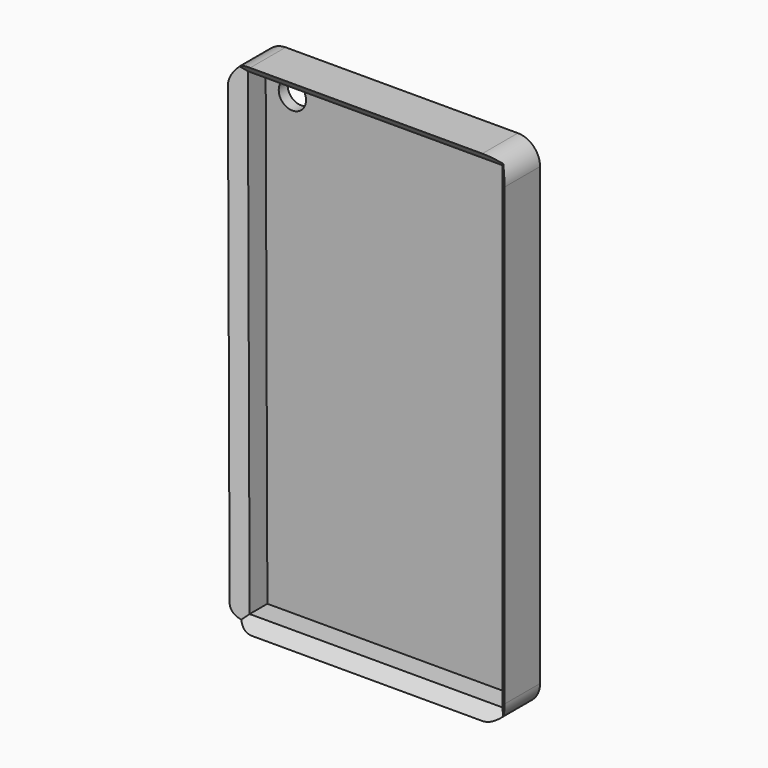
from build123d import *

# Parameters (mm, degrees)
F1_DEPTH     = 12.7
F2_T         = -2.54
F3_R         = 5.08
F4_T1_DEPTH  = 109.2192415341
F4_T6_DEPTH  = 70.8878458195
F4_T11_DEPTH = 71.2857341695
F4_T16_DEPTH = 135.3482654479
F4_T23_DEPTH = 70.8878458195
F4_S24_R     = 5.08
F4_T25_DEPTH = 37
F4_T29_DEPTH = 135.3482654479
F4_S30_R     = 5.08
F4_T31_DEPTH = 69
F4_T38_DEPTH = 122.283391113
F4_S39_R     = 5.08
F4_T40_DEPTH = 63
F4_T44_DEPTH = 83.9519953984
F4_S45_R     = 5.08
F4_T46_DEPTH = 44
F4_T53_DEPTH = 84.3498837483
F4_S54_R     = 5.08
F4_T55_DEPTH = 44
F4_T59_DEPTH = 122.283391113
F4_S60_R     = 5.08
F4_T61_DEPTH = 63
F4_T68_DEPTH = 71.2857341695
F4_S69_R     = 5.08
F4_T70_DEPTH = 37
F4_T74_DEPTH = 135.3482654479
F4_S75_R     = 5.08
F4_T76_DEPTH = 69
F5_R         = 3.1205414485
F6_DEPTH     = 25.4


# Not quite as in the source:
# - a fillet or chamfer that OpenCascade refuses, or shapes differently, is made with other operations: its cross-section is extruded or revolved along the edge and cut away or added


with BuildPart() as f1:
    # F0 (on Front) → F1 (new body)
    with BuildSketch(Plane.XZ):
        Polygon((-76.0919898748, 56.9143295288), (-75.6755949615, -57.3849120053), (-12.7811351476, -57.3849120053), (-12.7811351476, 56.9143295288), align=None)
    extrude(amount=F1_DEPTH)

    # F2
    f2_openings = [f1.faces().sort_by_distance(p)[0] for p in [
        (-44.332578, -12.7, -0.172439),
    ]]
    offset(amount=F2_T, openings=f2_openings)

    # F3
    f3_edges = [f1.edges().sort_by_distance(p)[0] for p in [
        (-12.781135, -6.35, 56.91433),
        (-76.09199, -6.35, 56.91433),
        (-12.781135, -6.35, -57.384912),
        (-75.675595, -6.35, -57.384912),
    ]]
    fillet(f3_edges, radius=F3_R)

    # F4: chamfer of 5.08 on 4 edges, made by hand

    # F4_s2 → F4_t1 (cut)
    with BuildSketch(Plane.XY.offset(-54.8449120053)):
        Polygon((-10.2411351476, -12.7), (-15.3211351476, -7.62), (-15.3211351476, -12.7), align=None)
    extrude(amount=F4_T1_DEPTH, mode=Mode.SUBTRACT)


with BuildPart() as f4_tool4:
    # F4_s5 → F4_t6 (new body)
    with BuildSketch(Plane.YZ.offset(-86.2089809671)):
        Polygon((-12.7, -59.9249120053), (-7.62, -54.8449120053), (-12.7, -54.8449120053), align=None)
    extrude(amount=F4_T6_DEPTH)

    split(bisect_by=Plane(origin=(-73.3436593453, 0, -0.2671927326), x_dir=(0, 1, 0), z_dir=(0.9999933643, 0, 0.0036430001)), keep=Keep.TOP)


with BuildPart() as f1_1:
    add(f1.part)

    # F4_t3: cut F4_tool4
    add(f4_tool4.part, mode=Mode.SUBTRACT)


with BuildPart() as f4_tool9:
    # F4_s10 → F4_t11 (new body)
    with BuildSketch(Plane.YZ.offset(-15.3211351476)):
        Polygon((-12.7, 59.4543295288), (-7.62, 54.3743295288), (-12.7, 54.3743295288), align=None)
    extrude(amount=-F4_T11_DEPTH)

    split(bisect_by=Plane(origin=(-73.3436593453, 0, -0.2671927326), x_dir=(0, 1, 0), z_dir=(0.9999933643, 0, 0.0036430001)), keep=Keep.TOP)


with BuildPart() as f1_2:
    add(f1_1.part)

    # F4_t8: cut F4_tool9
    add(f4_tool9.part, mode=Mode.SUBTRACT)


with BuildPart() as f4_tool14:
    # F4_s15 → F4_t16 (new body)
    with BuildSketch(Plane(origin=(-0.2466530914, 0, 67.7055851499), x_dir=(0, 1, 0), z_dir=(0.0036430001, 0, -0.9999933643))):
        Polygon((-12.7, -78.4241460385), (-7.62, -73.3441460385), (-12.7, -73.3441460385), align=None)
    extrude(amount=F4_T16_DEPTH)

    split(bisect_by=Plane.XY.offset(54.3743295288), keep=Keep.BOTTOM)

    split(bisect_by=Plane.XY.offset(-54.8449120053), keep=Keep.TOP)


with BuildPart() as f1_3:
    add(f1_2.part)

    # F4_t13: cut F4_tool14
    add(f4_tool14.part, mode=Mode.SUBTRACT)


with BuildPart() as f4_tool21:
    # F4_s22 → F4_t23 (new body)
    with BuildSketch(Plane.YZ.offset(-86.2089809671)):
        Polygon((-12.7, -59.9249120053), (-7.62, -54.8449120053), (-12.7, -54.8449120053), align=None)
    extrude(amount=F4_T23_DEPTH)

    # F4_s24 → F4_t25 (intersect, symmetric)
    with BuildSketch(Plane.XZ.offset(10.2)):
        with Locations((-70.614067815, -52.3049120053)):
            Circle(F4_S24_R)
    extrude(amount=F4_T25_DEPTH, both=True, mode=Mode.INTERSECT)

    split(bisect_by=Plane(origin=(-73.3436593453, 0, -0.2671927326), x_dir=(0, 1, 0), z_dir=(-0.9999933643, 0, -0.0036430001)), keep=Keep.TOP)


with BuildPart() as f4_tool27:
    # F4_s28 → F4_t29 (new body)
    with BuildSketch(Plane(origin=(-0.2466530914, 0, 67.7055851499), x_dir=(0, 1, 0), z_dir=(0.0036430001, 0, -0.9999933643))):
        Polygon((-12.7, -78.4241460385), (-7.62, -73.3441460385), (-12.7, -73.3441460385), align=None)
    extrude(amount=F4_T29_DEPTH)

    # F4_s30 → F4_t31 (intersect, symmetric)
    with BuildSketch(Plane.XZ.offset(10.2)):
        with Locations((-70.614067815, -52.3049120053)):
            Circle(F4_S30_R)
    extrude(amount=F4_T31_DEPTH, both=True, mode=Mode.INTERSECT)

    split(bisect_by=Plane.XY.offset(-54.8449120053), keep=Keep.BOTTOM)


with BuildPart() as f4_tool21_1:
    add(f4_tool21.part)

    # F4_t33: intersect F4_tool27
    add(f4_tool27.part, mode=Mode.INTERSECT)


with BuildPart() as f1_4:
    add(f1_3.part)

    # F4_t19: cut F4_tool21
    add(f4_tool21_1.part, mode=Mode.SUBTRACT)


with BuildPart() as f4_tool36:
    # F4_s37 → F4_t38 (new body)
    with BuildSketch(Plane.XY.offset(-67.9090615842)):
        Polygon((-10.2411351476, -12.7), (-15.3211351476, -7.62), (-15.3211351476, -12.7), align=None)
    extrude(amount=F4_T38_DEPTH)

    # F4_s39 → F4_t40 (intersect, symmetric)
    with BuildSketch(Plane.XZ.offset(10.2)):
        with Locations((-17.8611351476, -52.3049120053)):
            Circle(F4_S39_R)
    extrude(amount=F4_T40_DEPTH, both=True, mode=Mode.INTERSECT)

    split(bisect_by=Plane.XY.offset(-54.8449120053), keep=Keep.BOTTOM)


with BuildPart() as f4_tool42:
    # F4_s43 → F4_t44 (new body)
    with BuildSketch(Plane.YZ.offset(-86.2089809671)):
        Polygon((-12.7, -59.9249120053), (-7.62, -54.8449120053), (-12.7, -54.8449120053), align=None)
    extrude(amount=F4_T44_DEPTH)

    # F4_s45 → F4_t46 (intersect, symmetric)
    with BuildSketch(Plane.XZ.offset(10.2)):
        with Locations((-17.8611351476, -52.3049120053)):
            Circle(F4_S45_R)
    extrude(amount=F4_T46_DEPTH, both=True, mode=Mode.INTERSECT)

    split(bisect_by=Plane.YZ.offset(-15.3211351476), keep=Keep.TOP)


with BuildPart() as f4_tool36_1:
    add(f4_tool36.part)

    # F4_t48: intersect F4_tool42
    add(f4_tool42.part, mode=Mode.INTERSECT)


with BuildPart() as f1_5:
    add(f1_4.part)

    # F4_t34: cut F4_tool36
    add(f4_tool36_1.part, mode=Mode.SUBTRACT)


with BuildPart() as f4_tool51:
    # F4_s52 → F4_t53 (new body)
    with BuildSketch(Plane.YZ.offset(-2.2569855688)):
        Polygon((-12.7, 59.4543295288), (-7.62, 54.3743295288), (-12.7, 54.3743295288), align=None)
    extrude(amount=-F4_T53_DEPTH)

    # F4_s54 → F4_t55 (intersect, symmetric)
    with BuildSketch(Plane.XZ.offset(10.2)):
        with Locations((-17.8611351476, 51.8343295288)):
            Circle(F4_S54_R)
    extrude(amount=F4_T55_DEPTH, both=True, mode=Mode.INTERSECT)

    split(bisect_by=Plane.YZ.offset(-15.3211351476), keep=Keep.TOP)


with BuildPart() as f4_tool57:
    # F4_s58 → F4_t59 (new body)
    with BuildSketch(Plane.XY.offset(-54.8449120053)):
        Polygon((-10.2411351476, -12.7), (-15.3211351476, -7.62), (-15.3211351476, -12.7), align=None)
    extrude(amount=F4_T59_DEPTH)

    # F4_s60 → F4_t61 (intersect, symmetric)
    with BuildSketch(Plane.XZ.offset(10.2)):
        with Locations((-17.8611351476, 51.8343295288)):
            Circle(F4_S60_R)
    extrude(amount=F4_T61_DEPTH, both=True, mode=Mode.INTERSECT)

    split(bisect_by=Plane.XY.offset(54.3743295288), keep=Keep.TOP)


with BuildPart() as f4_tool51_1:
    add(f4_tool51.part)

    # F4_t63: intersect F4_tool57
    add(f4_tool57.part, mode=Mode.INTERSECT)


with BuildPart() as f1_6:
    add(f1_5.part)

    # F4_t49: cut F4_tool51
    add(f4_tool51_1.part, mode=Mode.SUBTRACT)


with BuildPart() as f4_tool66:
    # F4_s67 → F4_t68 (new body)
    with BuildSketch(Plane.YZ.offset(-15.3211351476)):
        Polygon((-12.7, 59.4543295288), (-7.62, 54.3743295288), (-12.7, 54.3743295288), align=None)
    extrude(amount=-F4_T68_DEPTH)

    # F4_s69 → F4_t70 (intersect, symmetric)
    with BuildSketch(Plane.XZ.offset(10.2)):
        with Locations((-70.9934496016, 51.8343295288)):
            Circle(F4_S69_R)
    extrude(amount=F4_T70_DEPTH, both=True, mode=Mode.INTERSECT)

    split(bisect_by=Plane(origin=(-73.3436593453, 0, -0.2671927326), x_dir=(0, 1, 0), z_dir=(-0.9999933643, 0, -0.0036430001)), keep=Keep.TOP)


with BuildPart() as f4_tool72:
    # F4_s73 → F4_t74 (new body)
    with BuildSketch(Plane(origin=(-0.2466530914, 0, 67.7055851499), x_dir=(0, 1, 0), z_dir=(0.0036430001, 0, -0.9999933643))):
        Polygon((-12.7, -78.4241460385), (-7.62, -73.3441460385), (-12.7, -73.3441460385), align=None)
    extrude(amount=F4_T74_DEPTH)

    # F4_s75 → F4_t76 (intersect, symmetric)
    with BuildSketch(Plane.XZ.offset(10.2)):
        with Locations((-70.9934496016, 51.8343295288)):
            Circle(F4_S75_R)
    extrude(amount=F4_T76_DEPTH, both=True, mode=Mode.INTERSECT)

    split(bisect_by=Plane.XY.offset(54.3743295288), keep=Keep.TOP)


with BuildPart() as f4_tool66_1:
    add(f4_tool66.part)

    # F4_t78: intersect F4_tool72
    add(f4_tool72.part, mode=Mode.INTERSECT)


with BuildPart() as f1_7:
    add(f1_6.part)

    # F4_t64: cut F4_tool66
    add(f4_tool66_1.part, mode=Mode.SUBTRACT)

    # F5 (on face) → F6 (cut)
    with BuildSketch(Plane(origin=(0, 0, 0), x_dir=(-1, 0, 0), z_dir=(0, 1, 0))):
        with Locations((67.4311071634, 49.4907200336)):
            Circle(F5_R)
    extrude(amount=-F6_DEPTH, mode=Mode.SUBTRACT)


solid = f1_7.part
